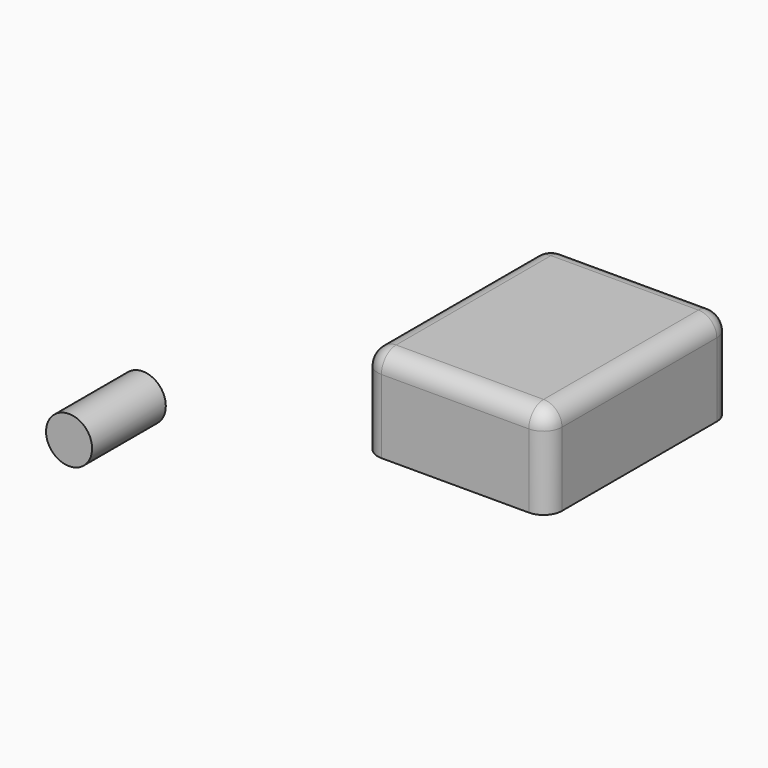
from build123d import *

# Parameters (mm, degrees)
F0_W         = 50.8
F0_H         = 63.5
F1_DEPTH     = 25.4
F2_R         = 6.35
F3_DEPTH     = 25.4
F4_R         = 5.08
F5_T1_DEPTH  = 33.02
F5_S5_W      = 5.08
F5_S5_H      = 5.08
F5_T6_DEPTH  = 5.08
F5_S11_W     = 5.08
F5_S11_H     = 5.08
F5_T12_DEPTH = 5.08
F5_S17_W     = 5.08
F5_S17_H     = 5.08
F5_T18_DEPTH = 5.08
F5_S23_W     = 5.08
F5_S23_H     = 5.08
F5_T24_DEPTH = 5.08


# Not quite as in the source:
# - a fillet or chamfer that OpenCascade refuses, or shapes differently, is made with other operations: its cross-section is extruded or revolved along the edge and cut away or added


with BuildPart() as f1:
    # F0 (on Top) → F1 (new body)
    with BuildSketch(Plane.XY):
        with Locations((25.4, 31.75)):
            Rectangle(F0_W, F0_H)
    extrude(amount=F1_DEPTH)

    # F4
    f4_edges = [f1.edges().sort_by_distance(p)[0] for p in [
        (25.4, 0, 25.4),
        (50.8, 31.75, 25.4),
        (25.4, 63.5, 25.4),
        (0, 31.75, 25.4),
    ]]
    fillet(f4_edges, radius=F4_R)

    # F5: fillet of radius 5.08 on 4 edges, made by hand

    # F5_s2 → F5_t1 (cut)
    with BuildSketch(Plane.XY.offset(-12.7)):
        with BuildLine():
            ThreePointArc((0, 5.08), (1.4878975516, 1.4878975516), (5.08, 0))
            Line((5.08, 0), (0, 0))
            Line((0, 0), (0, 5.08))
        make_face()
        with BuildLine():
            ThreePointArc((45.72, 0), (49.3121024484, 1.4878975516), (50.8, 5.08))
            Line((50.8, 5.08), (50.8, 0))
            Line((50.8, 0), (45.72, 0))
        make_face()
        with BuildLine():
            ThreePointArc((45.72, 63.5), (49.3121024484, 62.0121024484), (50.8, 58.42))
            Line((50.8, 58.42), (50.8, 63.5))
            Line((50.8, 63.5), (45.72, 63.5))
        make_face()
        with BuildLine():
            ThreePointArc((0, 58.42), (1.4878975516, 62.0121024484), (5.08, 63.5))
            Line((5.08, 63.5), (0, 63.5))
            Line((0, 63.5), (0, 58.42))
        make_face()
    extrude(amount=F5_T1_DEPTH, mode=Mode.SUBTRACT)


with BuildPart() as f3:
    # F2 (on Front) → F3 (new body)
    with BuildSketch(Plane.XZ):
        with Locations((-60.7038587332, -6.6716084257)):
            Circle(F2_R)
    extrude(amount=F3_DEPTH)


with BuildPart() as f5_tool4:
    # F5_s5 → F5_t6 (new body)
    with BuildSketch(Plane.YZ.offset(5.08)):
        with Locations((60.96, 22.86)):
            Rectangle(F5_S5_W, F5_S5_H)
    extrude(amount=-F5_T6_DEPTH)

    # F5_s7 → F5_t8 (revolve, cut)
    with BuildSketch(Plane(origin=(5.08, 58.42, 20.32), x_dir=(0, -0.7071067812, -0.7071067812), z_dir=(0, 0.7071067812, -0.7071067812))):
        with BuildLine():
            ThreePointArc((0, -5.08), (5.08, 0), (0, 5.08))
            Line((0, 5.08), (0, -5.08))
        make_face()
    revolve(axis=Axis((5.08, 58.42, 20.32), (-1, 0, 0)), mode=Mode.SUBTRACT)


with BuildPart() as f1_1:
    add(f1.part)

    # F5_t3: cut F5_tool4
    add(f5_tool4.part, mode=Mode.SUBTRACT)


with BuildPart() as f5_tool10:
    # F5_s11 → F5_t12 (new body)
    with BuildSketch(Plane.XZ.offset(-58.42)):
        with Locations((48.26, 22.86)):
            Rectangle(F5_S11_W, F5_S11_H)
    extrude(amount=-F5_T12_DEPTH)

    # F5_s13 → F5_t14 (revolve, cut)
    with BuildSketch(Plane(origin=(45.72, 58.42, 20.32), x_dir=(-0.7071067812, 0, -0.7071067812), z_dir=(0.7071067812, 0, -0.7071067812))):
        with BuildLine():
            ThreePointArc((0, -5.08), (5.08, 0), (0, 5.08))
            Line((0, 5.08), (0, -5.08))
        make_face()
    revolve(axis=Axis((45.72, 58.42, 20.32), (0, 1, 0)), mode=Mode.SUBTRACT)


with BuildPart() as f1_2:
    add(f1_1.part)

    # F5_t9: cut F5_tool10
    add(f5_tool10.part, mode=Mode.SUBTRACT)


with BuildPart() as f5_tool16:
    # F5_s17 → F5_t18 (new body)
    with BuildSketch(Plane.XZ.offset(-5.08)):
        with Locations((48.26, 22.86)):
            Rectangle(F5_S17_W, F5_S17_H)
    extrude(amount=F5_T18_DEPTH)

    # F5_s19 → F5_t20 (revolve, cut)
    with BuildSketch(Plane(origin=(45.72, 5.08, 20.32), x_dir=(-0.7071067812, 0, -0.7071067812), z_dir=(-0.7071067812, 0, 0.7071067812))):
        with BuildLine():
            ThreePointArc((0, -5.08), (5.08, 0), (0, 5.08))
            Line((0, 5.08), (0, -5.08))
        make_face()
    revolve(axis=Axis((45.72, 5.08, 20.32), (0, -1, 0)), mode=Mode.SUBTRACT)


with BuildPart() as f1_3:
    add(f1_2.part)

    # F5_t15: cut F5_tool16
    add(f5_tool16.part, mode=Mode.SUBTRACT)


with BuildPart() as f5_tool22:
    # F5_s23 → F5_t24 (new body)
    with BuildSketch(Plane.YZ.offset(5.08)):
        with Locations((2.54, 22.86)):
            Rectangle(F5_S23_W, F5_S23_H)
    extrude(amount=-F5_T24_DEPTH)

    # F5_s25 → F5_t26 (revolve, cut)
    with BuildSketch(Plane(origin=(5.08, 5.08, 20.32), x_dir=(0, 0.7071067812, -0.7071067812), z_dir=(0, 0.7071067812, 0.7071067812))):
        with BuildLine():
            ThreePointArc((0, -5.08), (5.08, 0), (0, 5.08))
            Line((0, 5.08), (0, -5.08))
        make_face()
    revolve(axis=Axis((5.08, 5.08, 20.32), (-1, 0, 0)), mode=Mode.SUBTRACT)


with BuildPart() as f1_4:
    add(f1_3.part)

    # F5_t21: cut F5_tool22
    add(f5_tool22.part, mode=Mode.SUBTRACT)


solid = Compound([f3.part, f1_4.part])
